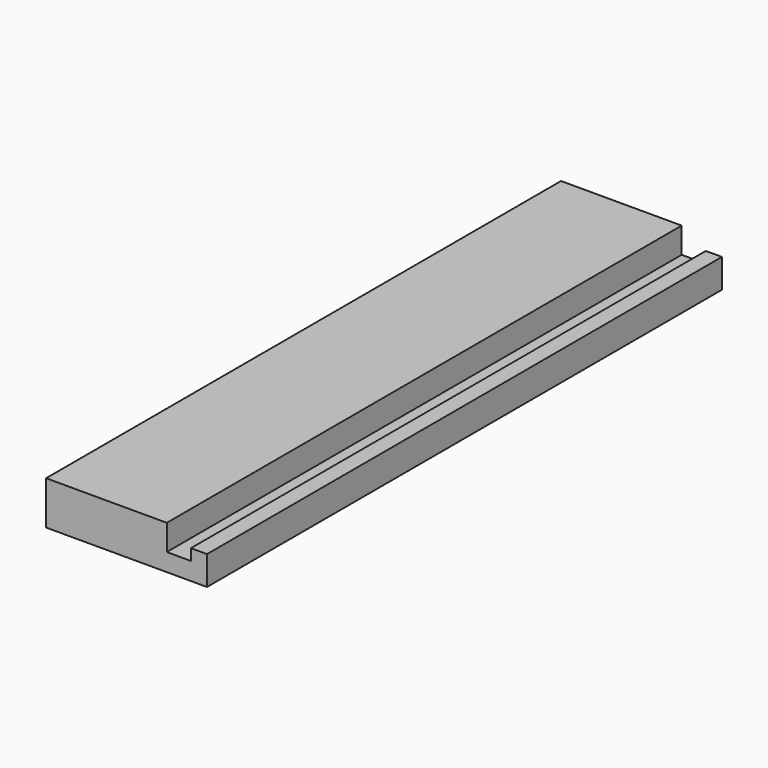
from build123d import *

# Parameters (mm, degrees)
F2_DEPTH = 27
F1_W     = 15
F1_H     = 400
F3_DEPTH = 11
F1_W_2   = 10
F4_DEPTH = 18


# Not quite as in the source:
# - a feature of the source that left no trace in its solid (it failed there, or was rolled back) is left out


with BuildPart() as f2:
    # F1 (on Top) → F2 (new body)
    with BuildSketch(Plane.XY):
        with BuildLine():
            Line((-1.25, 200), (-37.5, 200))
            Line((-37.5, 200), (-37.5, -200))
            Line((-37.5, -200), (37.5, -200))
            Line((37.5, -200), (37.5, 200))
            Line((37.5, 200), (1.25, 200))
            Line((1.25, 200), (1.25, -184.1316527028))
            ThreePointArc((1.25, -184.1316527028), (4.6636895265, -186.2250827824), (6, -190))
            ThreePointArc((6, -190), (-3.7749172176, -194.6636895265), (-1.25, -184.1316527028))
            Line((-1.25, -184.1316527028), (-1.25, 200))
        make_face()
        with BuildLine():
            Line((1.25, 200), (-1.25, 200))
            Line((-1.25, 200), (-1.25, -184.1316527028))
            ThreePointArc((-1.25, -184.1316527028), (0, -184), (1.25, -184.1316527028))
            Line((1.25, -184.1316527028), (1.25, 200))
        make_face()
        with BuildLine():
            ThreePointArc((1.25, -184.1316527028), (0, -184), (-1.25, -184.1316527028))
            ThreePointArc((-1.25, -184.1316527028), (-3.7749172176, -194.6636895265), (6, -190))
            ThreePointArc((6, -190), (4.6636895265, -186.2250827824), (1.25, -184.1316527028))
        make_face()
    extrude(amount=F2_DEPTH)

    # F1 (on Top) → F3 (join)
    with BuildSketch(Plane.XY):
        with Locations((45, 0)):
            Rectangle(F1_W, F1_H)
    extrude(amount=F3_DEPTH)

    # F1 (on Top) → F4 (join)
    with BuildSketch(Plane.XY):
        with Locations((57.5, 0)):
            Rectangle(F1_W_2, F1_H)
    extrude(amount=F4_DEPTH)


solid = f2.part
